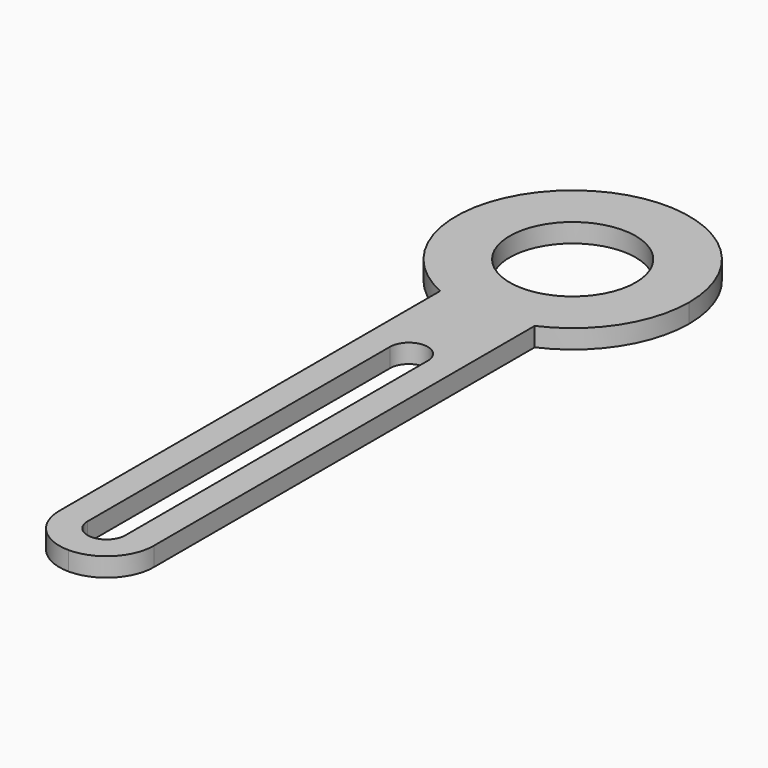
from build123d import *

# Parameters (mm, degrees)
F1_DEPTH = 3
F2_R     = 10
F3_DEPTH = 25
F4_R     = 7.49999
F6_DEPTH = 25


# Not quite as in the source:
# - a fillet or chamfer is up to 0.001 mm smaller than in the source, because OpenCascade refuses the exact size


with BuildPart() as f1:
    # F0 (on Top) → F1 (new body)
    with BuildSketch(Plane.XY):
        with BuildLine():
            Line((7.5, -16.9115345253), (7.5, 16.9115345253))
            ThreePointArc((7.5, 16.9115345253), (0, 18.5), (-7.5, 16.9115345253))
            Line((-7.5, 16.9115345253), (-7.5, -16.9115345253))
            ThreePointArc((-7.5, -16.9115345253), (0, -18.5), (7.5, -16.9115345253))
        make_face()
        with BuildLine():
            Line((-7.5, -16.9115345253), (-7.5, 16.9115345253))
            ThreePointArc((-7.5, 16.9115345253), (-18.5, 0), (-7.5, -16.9115345253))
        make_face()
        with BuildLine():
            ThreePointArc((7.5, -16.9115345253), (15.5080624193, -10.0871205009), (18.5, 0))
            ThreePointArc((18.5, 0), (15.5080624193, 10.0871205009), (7.5, 16.9115345253))
            Line((7.5, 16.9115345253), (7.5, -16.9115345253))
        make_face()
        with BuildLine():
            Line((7.5, -100), (7.5, -16.9115345253))
            ThreePointArc((7.5, -16.9115345253), (0, -18.5), (-7.5, -16.9115345253))
            Line((-7.5, -16.9115345253), (-7.5, -100))
            Line((-7.5, -100), (7.5, -100))
        make_face()
    extrude(amount=F1_DEPTH)

    # F2 (on face) → F3 (cut)
    with BuildSketch(Plane.XY.offset(3)):
        Circle(F2_R)
    extrude(amount=-F3_DEPTH, mode=Mode.SUBTRACT)

    # F4 (radius 7.5 in the source; OpenCascade refuses exactly that, so slightly less here)
    f4_edges = [f1.edges().sort_by_distance(p)[0] for p in [
        (7.5, -100, 1.5),
        (-7.5, -100, 1.5),
    ]]
    fillet(f4_edges, radius=F4_R)

    # F5 (on face) → F6 (cut)
    with BuildSketch(Plane.XY.offset(3)):
        with BuildLine():
            ThreePointArc((-3, -92.5), (0, -95.5), (3, -92.5))
            Line((3, -92.5), (3, -32.5))
            ThreePointArc((3, -32.5), (0, -29.5), (-3, -32.5))
            Line((-3, -32.5), (-3, -92.5))
        make_face()
    extrude(amount=-F6_DEPTH, mode=Mode.SUBTRACT)


solid = f1.part
